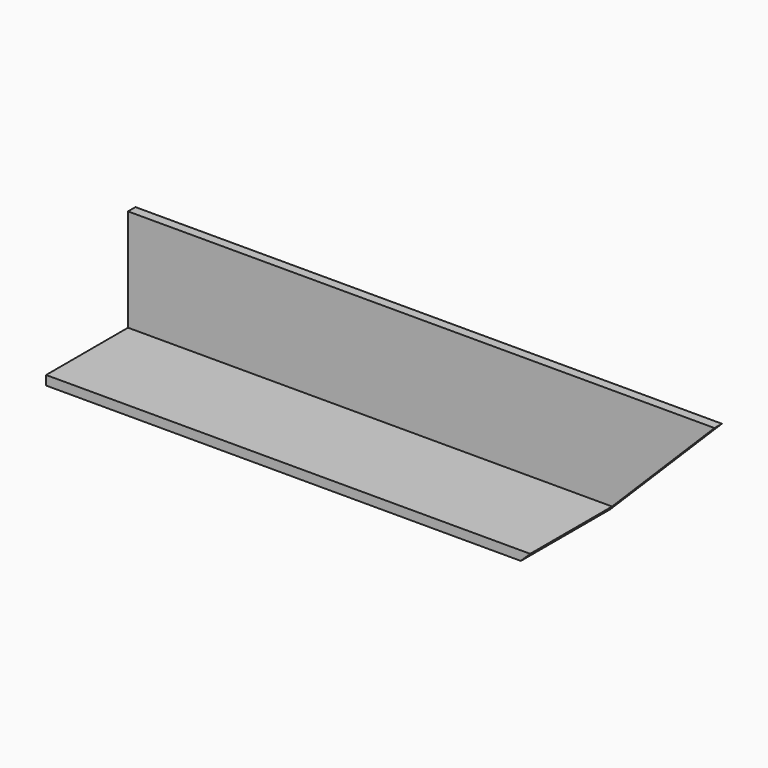
from build123d import *

# Parameters (mm, degrees)
F1_DEPTH = 6.35
F0_W     = 330.2
F0_H     = 6.35
F2_DEPTH = 76.2
F3_SIZE  = 6.34999


# Not quite as in the source:
# - a fillet or chamfer is up to 0.001 mm smaller than in the source, because OpenCascade refuses the exact size


with BuildPart() as f1:
    # F0 (on Front) → F1 (new body)
    with BuildSketch(Plane.XZ):
        Polygon((-278.9664838675, 77.2139622109), (-278.9664838675, 7.3639622109), (51.2335161325, 7.3639622109), (121.0835161325, 77.2139622109), align=None)
    extrude(amount=F1_DEPTH)

    # F0 (on Front) → F2 (join)
    with BuildSketch(Plane.XZ):
        with Locations((-113.8664838675, 4.1889622109)):
            Rectangle(F0_W, F0_H)
    extrude(amount=F2_DEPTH)

    # F3 (size 6.35 in the source; OpenCascade refuses exactly that, so slightly less here)
    f3_edges = [f1.edges().sort_by_distance(p)[0] for p in [
        (51.233516, -38.1, 1.013962),
    ]]
    chamfer(f3_edges, length=F3_SIZE)


solid = f1.part
